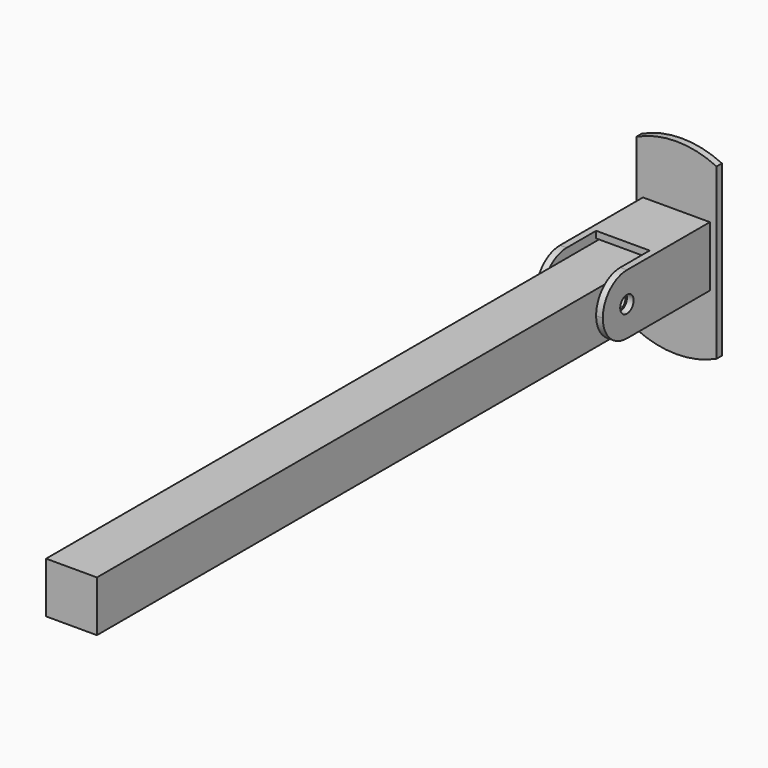
from build123d import *

# Parameters (mm, degrees)
F1_DEPTH  = 3.175
F3_DEPTH  = 31.75
F5_DEPTH  = 31.75
F6_R      = 14.28749
F8_D      = 7.9375
F8_DEPTH  = 50.8
F8_TIP    = 2.3846655818
F10_W     = 24.13
F10_H     = 24.13
F11_DEPTH = 355.6
F13_D     = 7.9375
F13_DEPTH = 50.8
F13_TIP   = 2.3846655818
F14_R     = 12.06499


# Not quite as in the source:
# - a fillet or chamfer is up to 0.001 mm smaller than in the source, because OpenCascade refuses the exact size


with BuildPart() as f1:
    # F0 (on Front) → F1 (new body)
    with BuildSketch(Plane.XZ):
        with BuildLine():
            Line((-19.05, 40.1609262841), (-19.05, -40.1609262841))
            ThreePointArc((-19.05, -40.1609262841), (0, -44.45), (19.05, -40.1609262841))
            Line((19.05, -40.1609262841), (19.05, 40.1609262841))
            ThreePointArc((19.05, 40.1609262841), (0, 44.45), (-19.05, 40.1609262841))
        make_face()
    extrude(amount=F1_DEPTH)

    # F2 (on face) → F3 (join)
    with BuildSketch(Plane.XZ.offset(3.175)):
        Polygon((-12.7, 12.7), (12.7, 12.7), (12.7, -12.7), (15.875, -12.7), (15.875, 15.875), (-15.875, 15.875), (-15.875, -12.7), (-12.7, -12.7), align=None)
    extrude(amount=F3_DEPTH)

    # F4 (on face) → F5 (join)
    with BuildSketch(Plane.XZ.offset(34.925)):
        Polygon((-12.7, 12.7), (-12.7, 15.875), (-15.875, 15.875), (-15.875, -12.7), (-12.7, -12.7), align=None)
        Polygon((15.875, 15.875), (12.7, 15.875), (12.7, 12.7), (12.7, -12.7), (15.875, -12.7), align=None)
    extrude(amount=F5_DEPTH)

    # F6 (radius 14.2875 in the source; OpenCascade refuses exactly that, so slightly less here)
    f6_edges = [f1.edges().sort_by_distance(p)[0] for p in [
        (-14.2875, -66.675, 15.875),
        (-14.2875, -66.675, -12.7),
        (14.2875, -66.675, -12.7),
        (14.2875, -66.675, 15.875),
    ]]
    fillet(f6_edges, radius=F6_R)

    # F8
    with Locations(Plane(origin=(-15.875, 0, 0), x_dir=(0, -1, 0), z_dir=(-1, 0, 0))):
        with Locations((52.3875, 1.5875)):
            Hole(F8_D / 2, depth=F8_DEPTH)
            with Locations((0, 0, -(F8_DEPTH + F8_TIP / 2))):  # 118° drill point
                Cone(0, F8_D / 2, F8_TIP, mode=Mode.SUBTRACT)


with BuildPart() as f11:
    # F10 (on offset) → F11 (new body)
    with BuildSketch(Plane.XZ.offset(6.35)):
        Rectangle(F10_W, F10_H)
    extrude(amount=F11_DEPTH)

    # F13
    with Locations(Plane(origin=(-12.065, 0, 0), x_dir=(0, -1, 0), z_dir=(-1, 0, 0))):
        with Locations((52.3875, 1.5875)):
            Hole(F13_D / 2, depth=F13_DEPTH)
            with Locations((0, 0, -(F13_DEPTH + F13_TIP / 2))):  # 118° drill point
                Cone(0, F13_D / 2, F13_TIP, mode=Mode.SUBTRACT)

    # F14 (radius 12.065 in the source; OpenCascade refuses exactly that, so slightly less here)
    f14_edges = [f11.edges().sort_by_distance(p)[0] for p in [
        (0, -6.35, 12.065),
        (0, -6.35, -12.065),
    ]]
    fillet(f14_edges, radius=F14_R)


solid = Compound([f1.part, f11.part])
